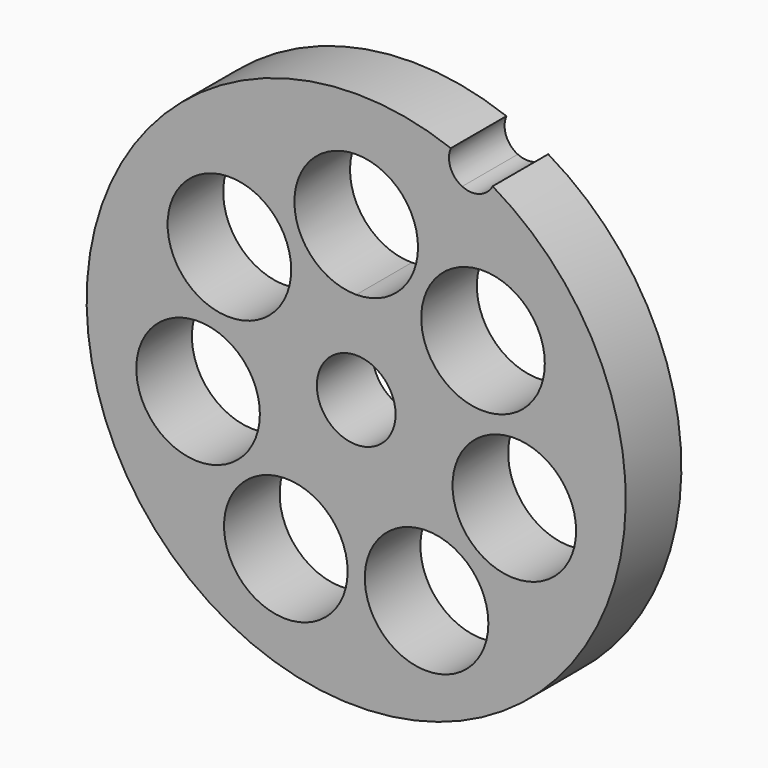
from build123d import *

# Parameters (mm, degrees)
F0_R     = 34.9
F0_R_2   = 5.1
F1_DEPTH = 9
F2_R     = 8
F3_DEPTH = 10
F5_DEPTH = 10


# Not quite as in the source:
# - a feature names something its author has since deleted; it is built from what else it names


with BuildPart() as f1:
    # F0 (on Front) → F1 (new body)
    with BuildSketch(Plane.XZ):
        Circle(F0_R)
        Circle(F0_R_2, mode=Mode.SUBTRACT)
    extrude(amount=-F1_DEPTH)

    # F2 (on Front) → F3 (cut)
    with BuildSketch(Plane.XZ):
        with Locations((-16.4184611318, 12.093285839)):
            Circle(F2_R)
        with Locations((-20.4734861558, -5.6729396131)):
            Circle(F2_R)
        with Locations((-9.1115585215, -19.920346226)):
            Circle(F2_R)
        with Locations((9.1115585215, -19.920346226)):
            Circle(F2_R)
        with Locations((20.4734861558, -5.6729396131)):
            Circle(F2_R)
        with BuildLine():
            ThreePointArc((8, 20), (5.6568542495, 25.6568542495), (0, 28))
            Line((0, 28), (0, 12))
            ThreePointArc((0, 12), (5.6568542495, 14.3431457505), (8, 20))
        make_face()
        with BuildLine():
            Line((0, 12), (0, 28))
            ThreePointArc((0, 28), (-8, 20), (0, 12))
        make_face()
        with Locations((16.4184611318, 12.093285839)):
            Circle(F2_R)
    extrude(amount=-F3_DEPTH, mode=Mode.SUBTRACT)

    # F4 (on face) → F5 (cut)
    with BuildSketch(Plane.XZ):
        with BuildLine():
            ThreePointArc((12.2493254993, 32.6797188607), (12.2053527551, 30.4437628813), (13.7203077268, 28.7986658698))
            Line((13.7203077268, 28.7986658698), (15.0106187983, 31.5070043529))
            ThreePointArc((15.0106187983, 31.5070043529), (13.6425787741, 32.1230453786), (12.2493254993, 32.6797188607))
        make_face()
        with BuildLine():
            Line((15.0106187983, 31.5070043529), (13.7203077268, 28.7986658698))
            ThreePointArc((13.7203077268, 28.7986658698), (15.9523075922, 28.6586324994), (17.6609971055, 30.1014813795))
            ThreePointArc((17.6609971055, 30.1014813795), (16.3509172571, 30.8327343071), (15.0106187983, 31.5070043529))
        make_face()
    extrude(amount=-F5_DEPTH, mode=Mode.SUBTRACT)


solid = f1.part
